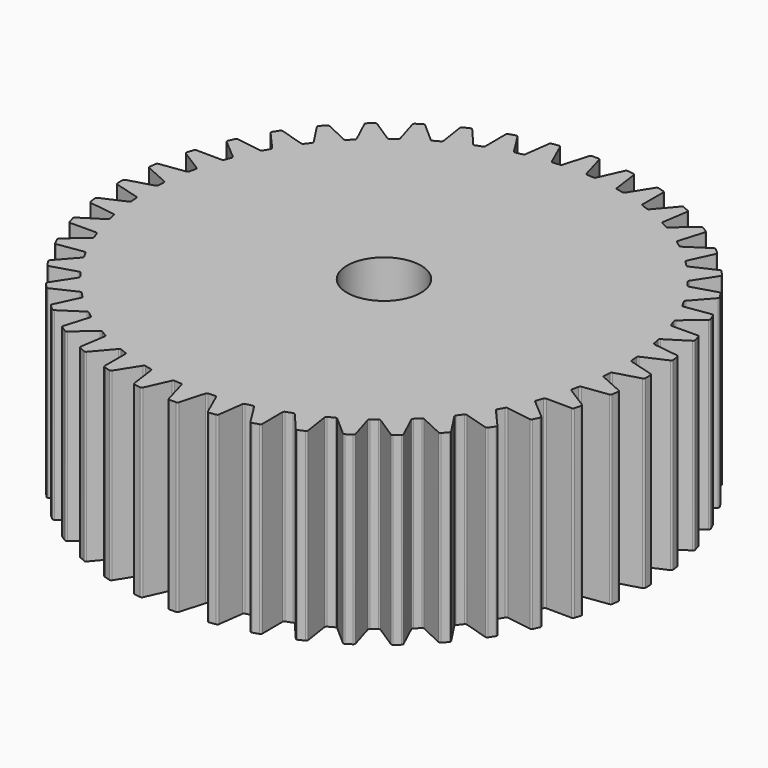
from build123d import *

# Parameters (mm, degrees)
F0_R            = 4
F1_DEPTH        = 20
F3_DEPTH        = 20.001
F3_COPIES_COUNT = 44


# Not quite as in the source:
# - a pattern or mirror of a feature is missing from the dataset's text; its kind, count and spacing are read off the source's solid


with BuildPart() as f1:
    # F0 (on Top) → F1 (new body)
    with BuildSketch(Plane.XY):
        Polygon((28.5942871124, -2.0451037768), (28.5942871124, 2.0451037768), (28.0121898859, 6.0936789151), (26.8598452538, 10.0182043234), (25.1607116297, 13.7387879818), (22.9493784744, 17.1796895362), (20.2708621539, 20.2708621539), (17.1796895362, 22.9493784744), (13.7387879818, 25.1607116297), (10.0182043234, 26.8598452538), (6.0936789151, 28.0121898859), (2.0451037768, 28.5942871124), (-2.0451037768, 28.5942871124), (-6.0936789151, 28.0121898859), (-10.0182043234, 26.8598452538), (-13.7387879818, 25.1607116297), (-17.1796895362, 22.9493784744), (-20.2708621539, 20.2708621539), (-22.9493784744, 17.1796895362), (-25.1607116297, 13.7387879818), (-26.8598452538, 10.0182043234), (-28.0121898859, 6.0936789151), (-28.5942871124, 2.0451037768), (-28.5942871124, -2.0451037768), (-28.0121898859, -6.0936789151), (-26.8598452538, -10.0182043234), (-25.1607116297, -13.7387879818), (-22.9493784744, -17.1796895362), (-20.2708621539, -20.2708621539), (-17.1796895362, -22.9493784744), (-13.7387879818, -25.1607116297), (-10.0182043234, -26.8598452538), (-6.0936789151, -28.0121898859), (-2.0451037768, -28.5942871124), (2.0451037768, -28.5942871124), (6.0936789151, -28.0121898859), (10.0182043234, -26.8598452538), (13.7387879818, -25.1607116297), (17.1796895362, -22.9493784744), (20.2708621539, -20.2708621539), (22.9493784744, -17.1796895362), (25.1607116297, -13.7387879818), (26.8598452538, -10.0182043234), (28.0121898859, -6.0936789151), align=None)
        Circle(F0_R, mode=Mode.SUBTRACT)
    extrude(amount=F1_DEPTH)

    # F2 (on face) → F3 (cut, through all)
    with BuildSketch(Plane.XY.offset(20)):
        with BuildLine():
            ThreePointArc((-3.7239037955, 28.3529121097), (-3.598895496, 28.330102036), (-3.5128610371, 28.2365849452))
            Line((-3.5128610371, 28.2365849452), (-2.3890576515, 25.7232212036))
            ThreePointArc((-2.3890576515, 25.7232212036), (-2.309213339, 25.6332616448), (-2.1922100241, 25.6053679045))
            Line((-2.1922100241, 25.6053679045), (-1.4741273053, 25.6567261942))
            ThreePointArc((-1.4741273053, 25.6567261942), (-1.3622846085, 25.7009873243), (-1.2960555761, 25.8013942549))
            Line((-1.2960555761, 25.8013942549), (-0.541379843, 28.4491094746))
            ThreePointArc((-0.541379843, 28.4491094746), (-0.4695299604, 28.5539186764), (-0.3490402772, 28.5942871124))
            Line((-0.3490402772, 28.5942871124), (-0.5, 28.5942871124))
            Line((-0.5, 28.5942871124), (-2.0451037768, 28.5942871124))
            Line((-2.0451037768, 28.5942871124), (-3.574480625, 28.3743959182))
            Line((-3.574480625, 28.3743959182), (-3.7239037955, 28.3529121097))
        make_face()
    f3 = extrude(amount=-F3_DEPTH, mode=Mode.SUBTRACT)

    # F3_copies: F3 ×44 about axis
    f3_copies_axis = Axis((0, 0, 0), (0, 0, 1))
    for i in range(1, F3_COPIES_COUNT):
        add(f3.rotate(f3_copies_axis, i * 360 / F3_COPIES_COUNT), mode=Mode.SUBTRACT)


solid = f1.part
